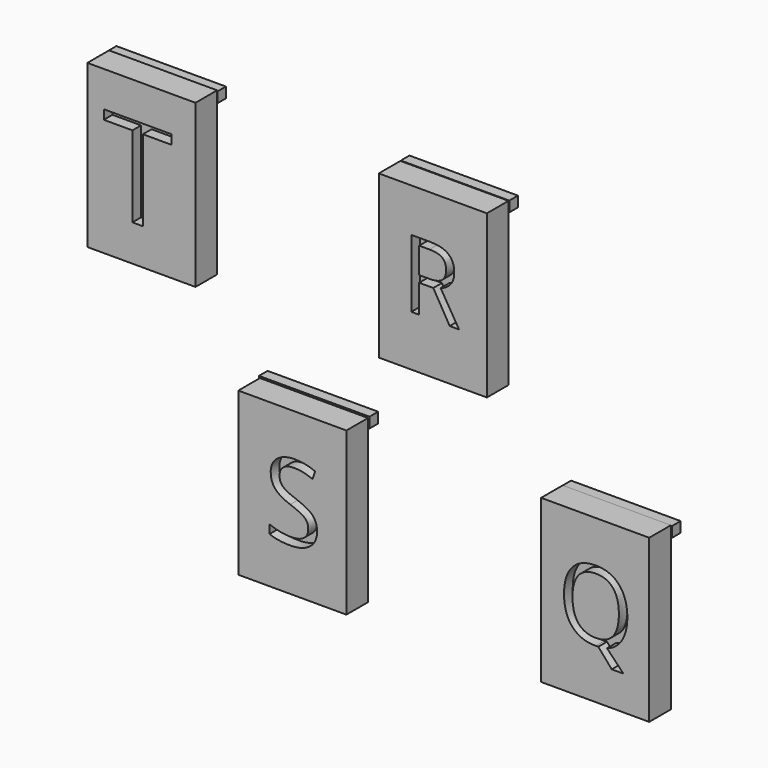
from build123d import *

# Parameters (mm, degrees)
F0_W           = 25.4
F0_H           = 38.1
F1_DEPTH       = 6.35
F2_R           = 3.81
F3_DEPTH       = 2.54
F5_TEXT_SIZE   = 22.6496835239
F5_TEXT_SIZE_2 = 22.2957822391
F5_TEXT_SIZE_3 = 24.773091233
F5_TEXT_SIZE_4 = 29.7277092209
F6_DEPTH       = 25.4
F7_W           = 25.730624795
F7_H           = 2.4505369365
F8_DEPTH       = 2.54
F7_W_2         = 25.4855751991
F7_W_3         = 25.7306285203
F7_W_4         = 25.9756827727
F7_H_2         = 2.4505350739


# Not quite as in the source:
# - Text() gives the source's letters only with a copy of the font that has no kerning and outlines rounded to 1/6400 em; it was checked with that copy


with BuildPart() as f1:
    # F0 (on Front) → F1 (new body)
    with BuildSketch(Plane.XZ):
        with Locations((-46.0602159804, 19.2970331914)):
            Rectangle(F0_W, F0_H)
    extrude(amount=F1_DEPTH)

    # F2 (on Front) → F3, piece 3 (join)
    with BuildSketch(Plane.XZ):
        with Locations((-40.9802159804, 18.0270331914)):
            Circle(F2_R)
        with Locations((-51.1402159804, 28.1870331914)):
            Circle(F2_R)
        with Locations((-51.1402159804, 18.0270331914)):
            Circle(F2_R)
        with Locations((-40.9802159804, 7.8670331914)):
            Circle(F2_R)
    extrude(amount=-F3_DEPTH)


with BuildPart() as f1b:
    # F0 (on Front) → F1, piece 2 (new body)
    with BuildSketch(Plane.XZ):
        with Locations((-10.603061258, -36.9614025138)):
            Rectangle(F0_W, F0_H)
    extrude(amount=F1_DEPTH)

    # F2 (on Front) → F3, piece 2 (join)
    with BuildSketch(Plane.XZ):
        with Locations((-5.523061258, -38.2314025138)):
            Circle(F2_R)
        with Locations((-15.683061258, -28.0714025138)):
            Circle(F2_R)
        with Locations((-5.523061258, -48.3914025138)):
            Circle(F2_R)
    extrude(amount=-F3_DEPTH)


with BuildPart() as f1c:
    # F0 (on Front) → F1, piece 3 (new body)
    with BuildSketch(Plane.XZ):
        with Locations((60.5514380593, -36.0065931796)):
            Rectangle(F0_W, F0_H)
    extrude(amount=F1_DEPTH)

    # F2 (on Front) → F3, piece 4 (join)
    with BuildSketch(Plane.XZ):
        with Locations((65.6314380593, -27.1165931796)):
            Circle(F2_R)
        with Locations((65.6314380593, -47.4365931796)):
            Circle(F2_R)
        with Locations((55.4714380593, -37.2765931796)):
            Circle(F2_R)
        with Locations((55.4714380593, -27.1165931796)):
            Circle(F2_R)
        with Locations((65.6314380593, -37.2765931796)):
            Circle(F2_R)
    extrude(amount=-F3_DEPTH)


with BuildPart() as f1d:
    # F0 (on Front) → F1, piece 4 (new body)
    with BuildSketch(Plane.XZ):
        with Locations((22.4085926682, 18.6961098781)):
            Rectangle(F0_W, F0_H)
    extrude(amount=F1_DEPTH)

    # F2 (on Front) → F3 (join)
    with BuildSketch(Plane.XZ):
        with Locations((27.4885926682, 7.2661098781)):
            Circle(F2_R)
        with Locations((27.4885926682, 17.4261098781)):
            Circle(F2_R)
        with Locations((27.4885926682, 27.5861098781)):
            Circle(F2_R)
        with Locations((17.3285926682, 17.4261098781)):
            Circle(F2_R)
    extrude(amount=-F3_DEPTH)


with BuildPart() as f6_tool:
    # F5 (on offset) → F6 (new body)
    with BuildSketch(Plane.XZ.offset(3.81)):
        with Locations((51.85360834, -43.1901142001)):
            Text('Q', F5_TEXT_SIZE, font='Open Sans', text_align=(TextAlign.LEFT, TextAlign.BOTTOM))
        with Locations((15.1611212641, 11.5938074887)):
            Text('R', F5_TEXT_SIZE_2, font='Open Sans', text_align=(TextAlign.LEFT, TextAlign.BOTTOM))
        with Locations((-17.1996122226, -45.7382043824)):
            Text('S', F5_TEXT_SIZE_3, font='Open Sans', text_align=(TextAlign.LEFT, TextAlign.BOTTOM))
        with Locations((-55.1661327481, 8.7909083813)):
            Text('T', F5_TEXT_SIZE_4, font='Open Sans', text_align=(TextAlign.LEFT, TextAlign.BOTTOM))
    extrude(amount=F6_DEPTH)


with BuildPart() as f1_1:
    add(f1.part)

    # F6: cut by f6_tool
    add(f6_tool.part, mode=Mode.SUBTRACT)

    # F7 (on Front) → F8, piece 3 (join)
    with BuildSketch(Plane.XZ):
        with Locations((-46.1926031858, 36.8805658072)):
            Rectangle(F7_W_3, F7_H)
    extrude(amount=-F8_DEPTH)


with BuildPart() as f1b_1:
    add(f1b.part)

    # F6: cut by f6_tool
    add(f6_tool.part, mode=Mode.SUBTRACT)

    # F7 (on Front) → F8, piece 4 (join)
    with BuildSketch(Plane.XZ):
        with Locations((-10.5373053811, -18.7466004863)):
            Rectangle(F7_W_4, F7_H_2)
    extrude(amount=-F8_DEPTH)


with BuildPart() as f1c_1:
    add(f1c.part)

    # F6: cut by f6_tool
    add(f6_tool.part, mode=Mode.SUBTRACT)

    # F7 (on Front) → F8 (join)
    with BuildSketch(Plane.XZ):
        with Locations((60.6507658958, -18.2564929128)):
            Rectangle(F7_W, F7_H)
    extrude(amount=-F8_DEPTH)


with BuildPart() as f1d_1:
    add(f1d.part)

    # F6: cut by f6_tool
    add(f6_tool.part, mode=Mode.SUBTRACT)

    # F7 (on Front) → F8, piece 2 (join)
    with BuildSketch(Plane.XZ):
        with Locations((22.5449316204, 36.6355124861)):
            Rectangle(F7_W_2, F7_H)
    extrude(amount=-F8_DEPTH)


solid = Compound([f1_1.part, f1b_1.part, f1c_1.part, f1d_1.part])
